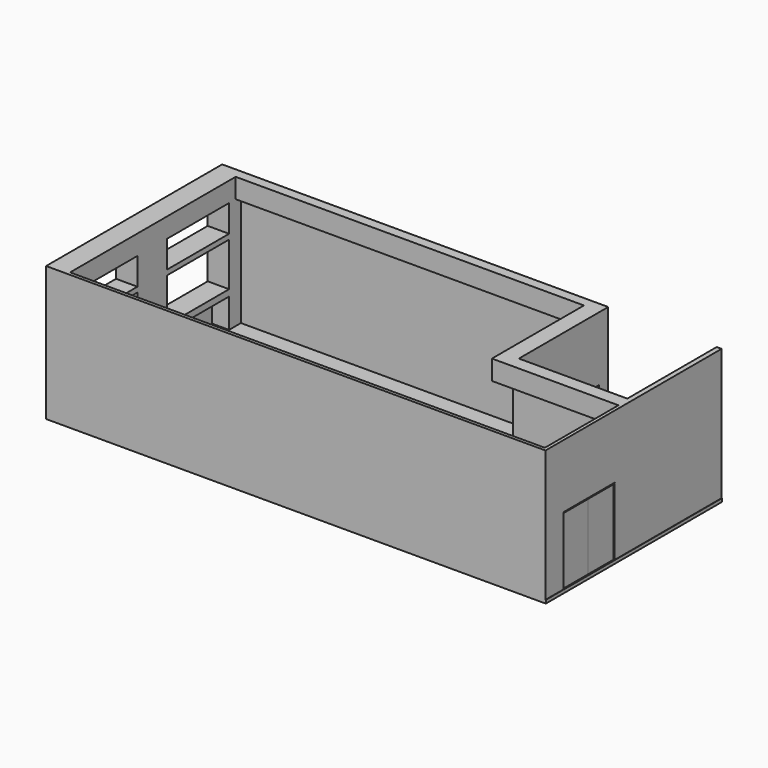
from build123d import *

# Parameters (mm, degrees)
F1_DEPTH       = 14500
F2_W           = 6700
F2_H           = 4100
F3_DEPTH       = 100
F4_W           = 3500
F4_H           = 4100
F5_DEPTH       = 3500
F6_W           = 3300
F6_H           = 3300
F7_DEPTH       = 4000
F8_W           = 3300
F8_H           = 4000
F9_DEPTH       = 300
F11_DEPTH      = 60
F11_DEPTH_BACK = 60
F13_DEPTH      = 30
F13_DEPTH_BACK = 30
F16_DEPTH      = 50
F17_W          = 6700
F17_H          = 4100
F17_W_2        = 1980
F17_H_2        = 2070
F18_DEPTH      = 50
F18_DEPTH_BACK = 50
F20_DEPTH      = 100
F21_W          = 40
F21_H          = 949
F22_DEPTH      = 2030
F23_W          = 6700
F23_H          = 100
F24_DEPTH      = 10
F26_DEPTH      = 10
F26_DEPTH_BACK = 110
F28_DEPTH      = 100
F29_W          = 40
F29_H          = 950
F30_DEPTH      = 2030
F31_W          = 2362.5
F31_H          = 1330
F32_DEPTH      = 100
F33_W          = 2362.5
F33_H          = 825
F34_DEPTH      = 100
F35_W          = 6700
F35_H          = 4100
F35_W_2        = 2362.5
F35_H_2        = 1330
F35_H_3        = 825
F36_DEPTH      = 35
F37_W          = 6700
F37_H          = 4100
F37_W_2        = 2362.5
F37_H_2        = 1330
F37_H_3        = 825
F38_DEPTH      = 515
F39_W          = 2362.5
F39_H          = 895
F40_DEPTH      = 515
F41_W          = 400
F41_H          = 600
F42_DEPTH      = 3700
F43_W          = 300
F43_H          = 600
F44_DEPTH      = 3450
F45_W          = 200
F45_H          = 600
F46_DEPTH      = 10600
F47_W          = 400
F47_H          = 250
F48_DEPTH      = 3400
F49_W          = 1550
F49_H          = 1100
F50_DEPTH      = 100


with BuildPart() as f1:
    # F0 (on Right) → F1 (new body)
    with BuildSketch(Plane.YZ):
        Polygon((6500, 0), (0, 0), (0, 4000), (-100, 4000), (-100, -100), (6600, -100), (6600, 4000), (6500, 4000), align=None)
    extrude(amount=F1_DEPTH)

    # F2 (on face) → F3 (join)
    with BuildSketch(Plane(origin=(0, 0, 0), x_dir=(0, -1, 0), z_dir=(-1, 0, 0))):
        with Locations((-3250, 1950)):
            Rectangle(F2_W, F2_H)
    extrude(amount=F3_DEPTH)

    # F4 (on face) → F5 (join)
    with BuildSketch(Plane.YZ.offset(14500)):
        with Locations((4850, 1950)):
            Rectangle(F4_W, F4_H)
    extrude(amount=-F5_DEPTH)

    # F6 (on face) → F7 (cut)
    with BuildSketch(Plane.XY.offset(4000)):
        with Locations((12750, 4850)):
            Rectangle(F6_W, F6_H)
    extrude(amount=-F7_DEPTH, mode=Mode.SUBTRACT)

    # F8 (on face) → F9 (cut)
    with BuildSketch(Plane.XZ.offset(-6500)):
        with Locations((12750, 2000)):
            Rectangle(F8_W, F8_H)
    extrude(amount=-F9_DEPTH, mode=Mode.SUBTRACT)

    # F15 (on face) → F16 (join)
    with BuildSketch(Plane.YZ.offset(14500)):
        Polygon((0, 4000), (0, 0), (560, 0), (560, 2070), (2540, 2070), (2540, 0), (3100, 0), (3100, 4000), align=None)
    extrude(amount=-F16_DEPTH)

    # F17 (on face) → F18 (join, two sides)
    with BuildSketch(Plane.YZ.offset(14500)) as f18_sk:
        with Locations((3250, 1950)):
            Rectangle(F17_W, F17_H)
        with Locations((1550, 1035)):
            Rectangle(F17_W_2, F17_H_2, mode=Mode.SUBTRACT)
    extrude(amount=F18_DEPTH)
    extrude(f18_sk.sketch, amount=-F18_DEPTH_BACK)

    # F19 (on face) → F20 (cut, through all)
    with BuildSketch(Plane(origin=(11000, 0, 0), x_dir=(0, -1, 0), z_dir=(-1, 0, 0))):
        Polygon((-3545, 0), (-3405, 0), (-3405, 2070), (-3445, 2070), (-4395, 2070), (-4435, 2070), (-4435, 0), align=None)
    extrude(amount=-F20_DEPTH, mode=Mode.SUBTRACT)

    # F23 (on face) → F24 (join, through all)
    with BuildSketch(Plane.YZ.offset(14550)):
        with Locations((3250, -50)):
            Rectangle(F23_W, F23_H)
    extrude(amount=F24_DEPTH)

    # F31 (on face) → F32 (cut, through all)
    with BuildSketch(Plane.YZ):
        with Locations((1381.25, 1755)):
            Rectangle(F31_W, F31_H)
        with Locations((4868.75, 1755)):
            Rectangle(F31_W, F31_H)
    extrude(amount=-F32_DEPTH, mode=Mode.SUBTRACT)

    # F33 (on face) → F34 (cut, through all)
    with BuildSketch(Plane.YZ):
        with Locations((1381.25, 2987.5)):
            Rectangle(F33_W, F33_H)
        with Locations((4868.75, 2987.5)):
            Rectangle(F33_W, F33_H)
    extrude(amount=-F34_DEPTH, mode=Mode.SUBTRACT)

    # F35 (on face) → F36 (join)
    with BuildSketch(Plane(origin=(-100, 0, 0), x_dir=(0, -1, 0), z_dir=(-1, 0, 0))):
        with Locations((-3250, 1950)):
            Rectangle(F35_W, F35_H)
        with Locations((-4868.75, 1755)):
            Rectangle(F35_W_2, F35_H_2, mode=Mode.SUBTRACT)
        with Locations((-1381.25, 1755)):
            Rectangle(F35_W_2, F35_H_2, mode=Mode.SUBTRACT)
        with Locations((-4868.75, 2987.5)):
            Rectangle(F35_W_2, F35_H_3, mode=Mode.SUBTRACT)
        with Locations((-1381.25, 2987.5)):
            Rectangle(F35_W_2, F35_H_3, mode=Mode.SUBTRACT)
    extrude(amount=F36_DEPTH)

    # F37 (on face) → F38 (join)
    with BuildSketch(Plane(origin=(-135, 0, 0), x_dir=(0, -1, 0), z_dir=(-1, 0, 0))):
        with Locations((-3250, 1950)):
            Rectangle(F37_W, F37_H)
        with Locations((-4868.75, 1755)):
            Rectangle(F37_W_2, F37_H_2, mode=Mode.SUBTRACT)
        with Locations((-1381.25, 1755)):
            Rectangle(F37_W_2, F37_H_2, mode=Mode.SUBTRACT)
        with Locations((-4868.75, 2987.5)):
            Rectangle(F37_W_2, F37_H_3, mode=Mode.SUBTRACT)
        with Locations((-1381.25, 2987.5)):
            Rectangle(F37_W_2, F37_H_3, mode=Mode.SUBTRACT)
    extrude(amount=F38_DEPTH)

    # F39 (on face) → F40 (cut)
    with BuildSketch(Plane.YZ):
        with Locations((1381.25, 447.5)):
            Rectangle(F39_W, F39_H)
        with Locations((4868.75, 447.5)):
            Rectangle(F39_W, F39_H)
    extrude(amount=-F40_DEPTH, mode=Mode.SUBTRACT)

    # F41 (on face) → F42 (join)
    with BuildSketch(Plane.XZ.offset(-6500)):
        with Locations((10800, 3700)):
            Rectangle(F41_W, F41_H)
    extrude(amount=F42_DEPTH)

    # F43 (on face) → F44 (join, through all)
    with BuildSketch(Plane.YZ.offset(11000)):
        with Locations((2950, 3700)):
            Rectangle(F43_W, F43_H)
    extrude(amount=F44_DEPTH)

    # F45 (on face) → F46 (join, through all)
    with BuildSketch(Plane(origin=(10600, 0, 0), x_dir=(0, -1, 0), z_dir=(-1, 0, 0))):
        with Locations((-6400, 3700)):
            Rectangle(F45_W, F45_H)
    extrude(amount=F46_DEPTH)

    # F47 (on face) → F48 (join, through all)
    with BuildSketch(Plane(origin=(0, 0, 3400), x_dir=(1, 0, 0), z_dir=(0, 0, -1))):
        with Locations((10800, -6375)):
            Rectangle(F47_W, F47_H)
    extrude(amount=F48_DEPTH)

    # F49 (on face) → F50 (cut, through all)
    with BuildSketch(Plane(origin=(11000, 0, 0), x_dir=(0, -1, 0), z_dir=(-1, 0, 0))):
        with Locations((-5465, 1500)):
            Rectangle(F49_W, F49_H)
    extrude(amount=-F50_DEPTH, mode=Mode.SUBTRACT)


with BuildPart() as f11:
    # F10 (on face) → F11 (new body, two sides)
    with BuildSketch(Plane.YZ.offset(14500)) as f11_sk:
        Polygon((2520, 2050), (2520, 0), (2540, 0), (2540, 2020), (2540, 2070), (1550, 2070), (560, 2070), (560, 2020), (560, 0), (580, 0), (580, 2050), align=None)
    extrude(amount=-F11_DEPTH)
    extrude(f11_sk.sketch, amount=F11_DEPTH_BACK)

    # F12 (on face) → F13 (join, two sides)
    with BuildSketch(Plane.YZ.offset(14500)) as f13_sk:
        Polygon((2500, 0), (2520, 0), (2520, 2050), (580, 2050), (580, 0), (600, 0), (600, 2030), (2500, 2030), align=None)
    extrude(amount=F13_DEPTH)
    extrude(f13_sk.sketch, amount=-F13_DEPTH_BACK)


with BuildPart() as f22:
    # F21 (on face) → F22 (new body, through all)
    with BuildSketch(Plane.XY):
        with Locations((14500, 2025.5)):
            Rectangle(F21_W, F21_H)
    extrude(amount=F22_DEPTH)


with BuildPart() as f22b:
    # F21 (on face) → F22, piece 2 (new body, through all)
    with BuildSketch(Plane.XY):
        with Locations((14500, 1074.5)):
            Rectangle(F21_W, F21_H)
    extrude(amount=F22_DEPTH)


with BuildPart() as f26:
    # F25 (on face) → F26 (new body, two sides)
    with BuildSketch(Plane(origin=(11000, 0, 0), x_dir=(0, -1, 0), z_dir=(-1, 0, 0))) as f26_sk:
        Polygon((-3405, 2070), (-4435, 2070), (-4435, 0), (-4415, 0), (-4415, 2050), (-3425, 2050), (-3425, 0), (-3405, 0), align=None)
    extrude(amount=F26_DEPTH)
    extrude(f26_sk.sketch, amount=-F26_DEPTH_BACK)

    # F27 (on face) → F28 (join)
    with BuildSketch(Plane(origin=(11000, 0, 0), x_dir=(0, -1, 0), z_dir=(-1, 0, 0))):
        Polygon((-4415, 2050), (-4415, 0), (-4395, 0), (-4395, 2030), (-3445, 2030), (-3445, 0), (-3425, 0), (-3425, 2050), align=None)
    extrude(amount=-F28_DEPTH)


with BuildPart() as f30:
    # F29 (on face) → F30 (new body, through all)
    with BuildSketch(Plane.XY):
        with Locations((11050, 3920)):
            Rectangle(F29_W, F29_H)
    extrude(amount=F30_DEPTH)


solid = Compound([f1.part, f11.part, f22.part, f22b.part, f26.part, f30.part])
